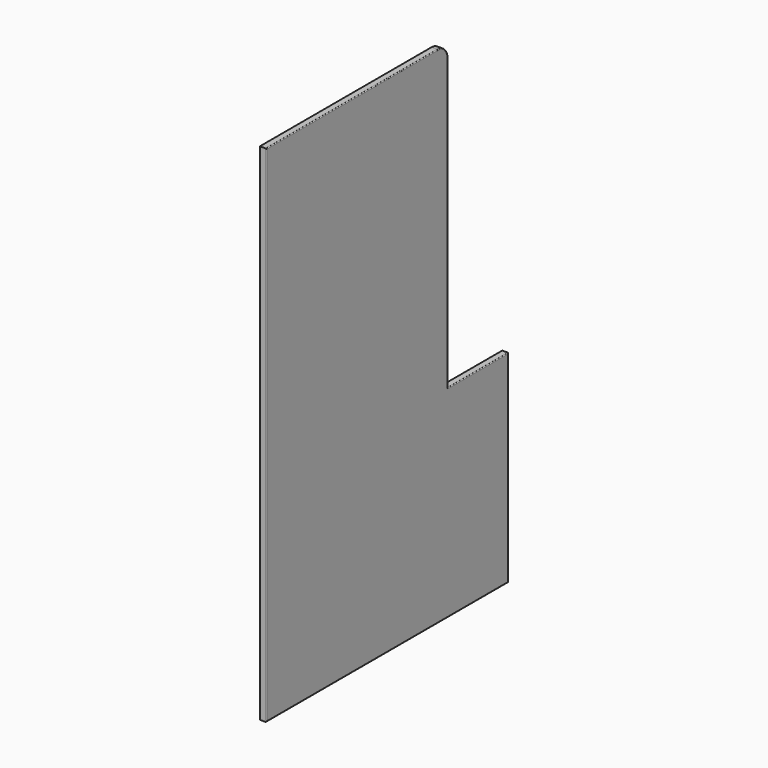
from build123d import *

# Parameters (mm, degrees)
F1_DEPTH    = 25
F2_R        = 3
F3_T1_DEPTH = 150
F3_T4_ANGLE = 90


# Not quite as in the source:
# - a fillet or chamfer that OpenCascade refuses, or shapes differently, is made with other operations: its cross-section is extruded or revolved along the edge and cut away or added


with BuildPart() as f1:
    # F0 (on Right) → F1 (new body)
    with BuildSketch(Plane.YZ):
        Polygon((0, 2000), (0, 0), (1200, 0), (1200, 800), (900, 800), (900, 2000), align=None)
    extrude(amount=F1_DEPTH)

    # F2
    f2_edges = [f1.edges().sort_by_distance(p)[0] for p in [
        (25, 0, 1000),
        (25, 600, 0),
        (25, 1200, 400),
        (25, 1050, 800),
        (25, 900, 1400),
        (25, 450, 2000),
    ]]
    fillet(f2_edges, radius=F2_R)

    # F3: fillet of radius 50 on 1 edges, made by hand

    # F3_s2 → F3_t1 (cut)
    with BuildSketch(Plane.YZ.offset(-125)):
        with BuildLine():
            ThreePointArc((850, 2000), (885.3553390593, 1985.3553390593), (900, 1950))
            Line((900, 1950), (900, 2000))
            Line((900, 2000), (850, 2000))
        make_face()
    extrude(amount=F3_T1_DEPTH, mode=Mode.SUBTRACT)

    # F3_s3 → F3_t4 (revolve, cut)
    with BuildSketch(Plane.XY.offset(1950)):
        with BuildLine():
            ThreePointArc((25, 897), (24.1213203436, 899.1213203436), (22, 900))
            Line((22, 900), (25, 900))
            Line((25, 900), (25, 897))
        make_face()
    revolve(axis=Axis((25, 850, 1950), (1, 0, 0)), revolution_arc=F3_T4_ANGLE, mode=Mode.SUBTRACT)


solid = f1.part
